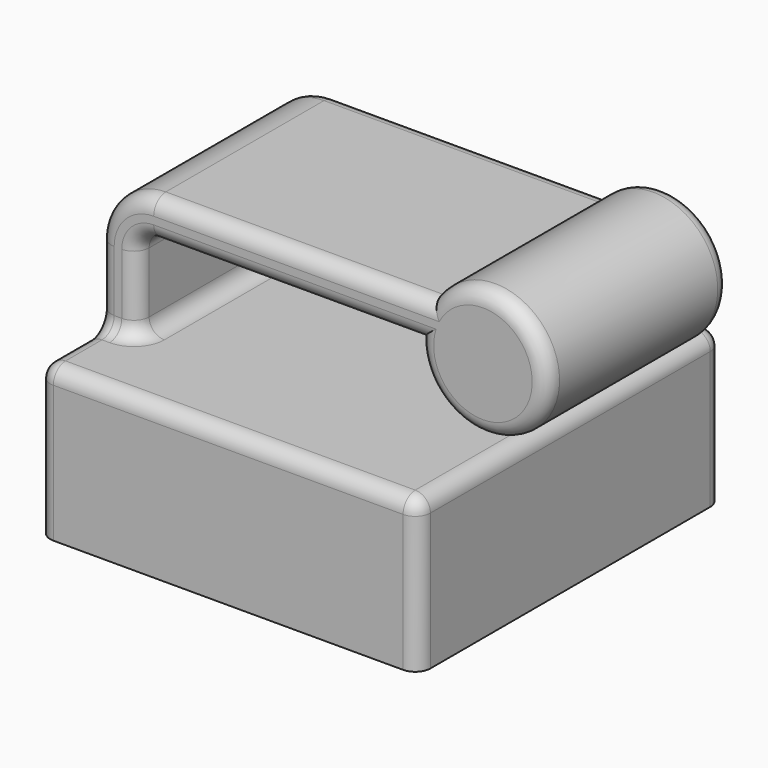
from build123d import *

# Parameters (mm, degrees)
F1_DEPTH = 63.5
F2_DEPTH = 38.1
F3_R     = 5.08


with BuildPart() as f1:
    # F0 (on Front) → F1 (new body, symmetric)
    with BuildSketch(Plane.XZ):
        Polygon((-63.5, 25.4), (-63.5, -25.4), (63.5, -25.4), (63.5, 25.4), (-50.8, 25.4), align=None)
    extrude(amount=F1_DEPTH, both=True)

    # F0 (on Front) → F2 (join, symmetric)
    with BuildSketch(Plane.XZ):
        with BuildLine():
            Line((-63.5, 50.8), (-63.5, 25.4))
            Line((-63.5, 25.4), (-50.8, 25.4))
            Line((-50.8, 25.4), (-50.8, 50.8))
            ThreePointArc((-50.8, 50.8), (-49.1655663717, 54.7458718322), (-45.2196945395, 56.3803054605))
            Line((-45.2196945395, 56.3803054605), (43.2454477532, 56.3803054605))
            ThreePointArc((43.2454477532, 56.3803054605), (44.3071420431, 63.0595111043), (47.3875670326, 69.0803054605))
            Line((47.3875670326, 69.0803054605), (-45.2196945395, 69.0803054605))
            ThreePointArc((-45.2196945395, 69.0803054605), (-58.1458224928, 63.7261279533), (-63.5, 50.8))
        make_face()
        with BuildLine():
            Line((64.7860094905, 69.0803054605), (47.3875670326, 69.0803054605))
            ThreePointArc((47.3875670326, 69.0803054605), (44.3071420431, 63.0595111043), (43.2454477532, 56.3803054605))
            Line((43.2454477532, 56.3803054605), (64.7860094905, 56.3803054605))
            Line((64.7860094905, 56.3803054605), (64.7860094905, 69.0803054605))
        make_face()
        with BuildLine():
            ThreePointArc((86.3265712278, 56.3803054605), (71.4652151342, 76.8591729079), (47.3875670326, 69.0803054605))
            Line((47.3875670326, 69.0803054605), (64.7860094905, 69.0803054605))
            Line((64.7860094905, 69.0803054605), (64.7860094905, 56.3803054605))
            Line((64.7860094905, 56.3803054605), (43.2454477532, 56.3803054605))
            ThreePointArc((43.2454477532, 56.3803054605), (64.7860094905, 34.8397437232), (86.3265712278, 56.3803054605))
        make_face()
    extrude(amount=F2_DEPTH, both=True)

    # F3
    f3_edges = [f1.edges().sort_by_distance(p)[0] for p in [
        (63.5, -63.5, 0),
        (-63.5, -63.5, 0),
        (63.5, 63.5, 0),
        (-63.5, 63.5, 0),
        (-58.145822, -38.1, 63.726128),
        (-63.5, -38.1, 38.1),
        (-57.15, -38.1, 25.4),
        (-50.8, -38.1, 38.1),
        (-49.165566, -38.1, 54.745872),
        (-0.987123, -38.1, 56.380305),
        (85.264877, -38.1, 49.7011),
        (1.083936, -38.1, 69.080305),
        (-58.145822, 38.1, 63.726128),
        (-63.5, 38.1, 38.1),
        (-57.15, 38.1, 25.4),
        (-50.8, 38.1, 38.1),
        (-49.165566, 38.1, 54.745872),
        (-0.987123, 38.1, 56.380305),
        (85.264877, 38.1, 49.7011),
        (1.083936, 38.1, 69.080305),
        (0, -63.5, 25.4),
        (63.5, 0, 25.4),
        (0, 63.5, 25.4),
        (-63.5, -50.8, 25.4),
        (-63.5, 50.8, 25.4),
        (-50.8, 0, 25.4),
    ]]
    fillet(f3_edges, radius=F3_R)


solid = f1.part
